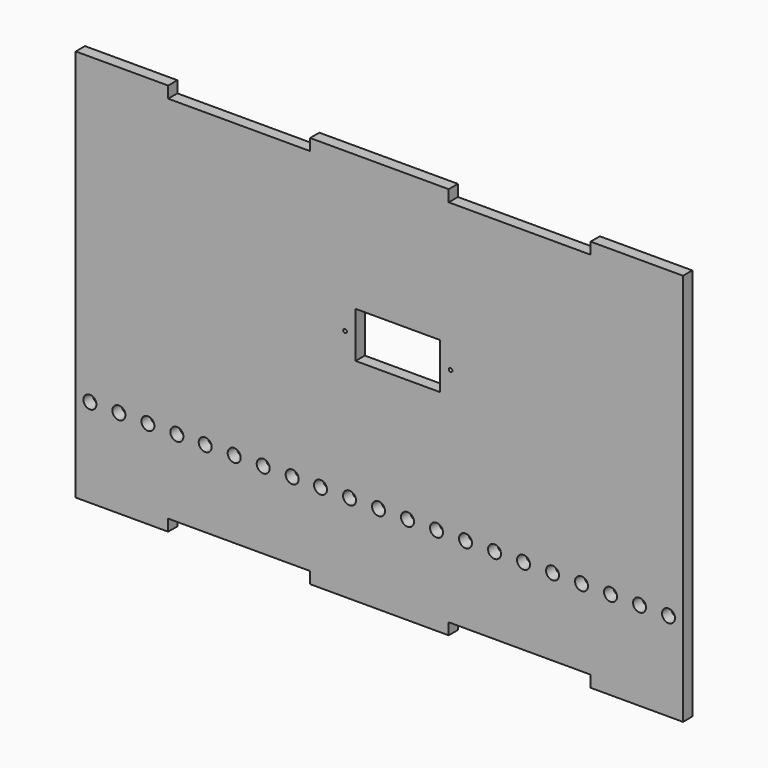
from build123d import *

# Parameters (mm, degrees)
F0_W     = 25.4
F0_H     = 3.175
F0_W_2   = 38.1
F0_R     = 1.7859375
F0_R_2   = 0.5
F1_DEPTH = 3.175


# Not quite as in the source:
# - a length typed as a fraction of an inch, garbled in the dataset ("3 / 203.2 mm" for 3/8 in), is restored


with BuildPart() as f1:
    # F0 (on Front) → F1 (new body)
    with BuildSketch(Plane.XZ):
        with Locations((-54.5774, 81.9875024)):
            Rectangle(F0_W, F0_H)
        with Locations((16.1738, 81.9875024)):
            Rectangle(F0_W_2, F0_H)
        with Locations((86.925, 81.9875024)):
            Rectangle(F0_W, F0_H)
        with Locations((86.925, -22.7875084)):
            Rectangle(F0_W, F0_H)
        with Locations((16.1738, -22.7875084)):
            Rectangle(F0_W_2, F0_H)
        with Locations((-54.5774, -22.7875084)):
            Rectangle(F0_W, F0_H)
        Polygon((-67.2774, 57.3229712169), (-67.2774, -21.2000084), (-41.8774, -21.2000084), (-2.8762, -21.2000084), (35.2238, -21.2000084), (74.225, -21.2000084), (99.625, -21.2000084), (99.625, 80.4000024), (74.225, 80.4000024), (35.2238, 80.4000024), (-2.8762, 80.4000024), (-41.8774, 80.4000024), (-67.2774, 80.4000024), align=None)
        with Locations((-63.3824, 0)):
            Circle(F0_R, mode=Mode.SUBTRACT)
        with Locations((-55.4124, 0)):
            Circle(F0_R, mode=Mode.SUBTRACT)
        with Locations((-47.4424, 0)):
            Circle(F0_R, mode=Mode.SUBTRACT)
        with Locations((-39.4724, 0)):
            Circle(F0_R, mode=Mode.SUBTRACT)
        with Locations((-31.7, 0)):
            Circle(F0_R, mode=Mode.SUBTRACT)
        with Locations((-23.73, 0)):
            Circle(F0_R, mode=Mode.SUBTRACT)
        with Locations((-15.76, 0)):
            Circle(F0_R, mode=Mode.SUBTRACT)
        with Locations((-7.79, 0)):
            Circle(F0_R, mode=Mode.SUBTRACT)
        Circle(F0_R, mode=Mode.SUBTRACT)
        with Locations((7.97, 0)):
            Circle(F0_R, mode=Mode.SUBTRACT)
        with Locations((15.94, 0)):
            Circle(F0_R, mode=Mode.SUBTRACT)
        with Locations((23.91, 0)):
            Circle(F0_R, mode=Mode.SUBTRACT)
        with Locations((31.88, 0)):
            Circle(F0_R, mode=Mode.SUBTRACT)
        with Locations((39.85, 0)):
            Circle(F0_R, mode=Mode.SUBTRACT)
        with Locations((47.82, 0)):
            Circle(F0_R, mode=Mode.SUBTRACT)
        with Locations((55.79, 0)):
            Circle(F0_R, mode=Mode.SUBTRACT)
        with Locations((63.76, 0)):
            Circle(F0_R, mode=Mode.SUBTRACT)
        with Locations((71.73, 0)):
            Circle(F0_R, mode=Mode.SUBTRACT)
        with Locations((79.7, 0)):
            Circle(F0_R, mode=Mode.SUBTRACT)
        with Locations((87.67, 0)):
            Circle(F0_R, mode=Mode.SUBTRACT)
        with Locations((95.64, 0)):
            Circle(F0_R, mode=Mode.SUBTRACT)
        with Locations((6.74, 40.005)):
            Circle(F0_R_2, mode=Mode.SUBTRACT)
        Polygon((9.64, 40.005), (9.64, 46.305), (15.94, 46.305), (32.84, 46.305), (32.84, 33.705), (15.94, 33.705), (9.64, 33.705), align=None, mode=Mode.SUBTRACT)
        with Locations((35.74, 40.005)):
            Circle(F0_R_2, mode=Mode.SUBTRACT)
    extrude(amount=F1_DEPTH)


solid = f1.part
